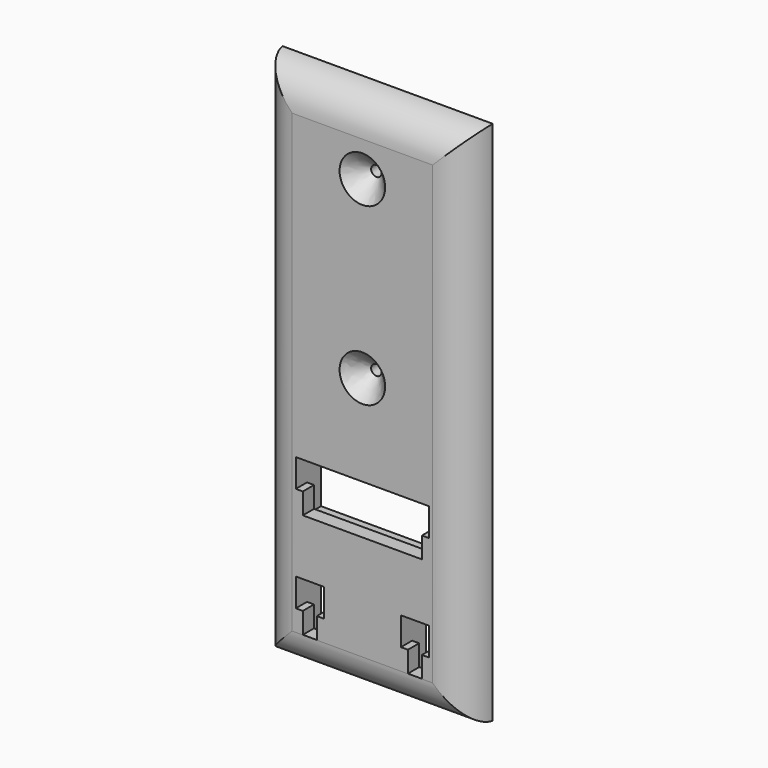
from build123d import *
from build123d import SkipClean  # not in build123d's __all__

# Parameters (mm, degrees)
F0_R        = 1.5
F1_DEPTH    = 5
F0_W        = 22
F0_H        = 2
F0_W_2      = 2
F0_H_2      = 6
F0_W_3      = 4
F2_DEPTH    = 4
F3_SIZE     = 5
F4_T1_DEPTH = 109.7493718553
F4_T3_DEPTH = 199.7493718553


# Not quite as in the source:
# - a fillet or chamfer that OpenCascade refuses, or shapes differently, is made with other operations: its cross-section is extruded or revolved along the edge and cut away or added
# - a feature names something its author has since deleted; it is built from what else it names


with BuildPart() as f1:
    # F0 (on Front) → F1 (new body)
    with BuildSketch(Plane.XZ):
        with BuildLine():
            Line((-30, 150), (-30, 80))
            Line((-30, 80), (-1.5, 80))
            ThreePointArc((-1.5, 80), (0, 81.5), (1.5, 80))
            Line((1.5, 80), (30, 80))
            Line((30, 80), (30, 150))
            Line((30, 150), (-30, 150))
        make_face()
        with Locations((0, 130)):
            Circle(F0_R, mode=Mode.SUBTRACT)
        with BuildLine():
            Line((-30, 0), (0, 0))
            Line((0, 0), (30, 0))
            Line((30, 0), (30, 80))
            Line((30, 80), (1.5, 80))
            ThreePointArc((1.5, 80), (0, 78.5), (-1.5, 80))
            Line((-1.5, 80), (-30, 80))
            Line((-30, 80), (-30, 0))
        make_face()
        Polygon((-11, 24), (-11, 16), (-11, 10), (-11, 8), (-13, 8), (-17, 8), (-19, 8), (-19, 10), (-19, 16), (-19, 24), align=None, mode=Mode.SUBTRACT)
        Polygon((19, 24), (19, 16), (19, 10), (19, 8), (17, 8), (13, 8), (11, 8), (11, 10), (11, 16), (11, 24), align=None, mode=Mode.SUBTRACT)
        Polygon((-19, 54), (-11, 54), (11, 54), (19, 54), (19, 46), (19, 40), (19, 38), (17, 38), (13, 38), (11, 38), (-11, 38), (-13, 38), (-17, 38), (-19, 38), (-19, 40), (-19, 46), (-19, 48), align=None, mode=Mode.SUBTRACT)
    extrude(amount=-F1_DEPTH)

    # F0 (on Front) → F2 (join)
    with BuildSketch(Plane.XZ):
        with BuildLine():
            Line((-30, 0), (0, 0))
            Line((0, 0), (30, 0))
            Line((30, 0), (30, 80))
            Line((30, 80), (1.5, 80))
            ThreePointArc((1.5, 80), (0, 78.5), (-1.5, 80))
            Line((-1.5, 80), (-30, 80))
            Line((-30, 80), (-30, 0))
        make_face()
        Polygon((-11, 24), (-11, 16), (-11, 10), (-11, 8), (-13, 8), (-17, 8), (-19, 8), (-19, 10), (-19, 16), (-19, 24), align=None, mode=Mode.SUBTRACT)
        Polygon((19, 24), (19, 16), (19, 10), (19, 8), (17, 8), (13, 8), (11, 8), (11, 10), (11, 16), (11, 24), align=None, mode=Mode.SUBTRACT)
        Polygon((-19, 54), (-11, 54), (11, 54), (19, 54), (19, 46), (19, 40), (19, 38), (17, 38), (13, 38), (11, 38), (-11, 38), (-13, 38), (-17, 38), (-19, 38), (-19, 40), (-19, 46), (-19, 48), align=None, mode=Mode.SUBTRACT)
        with BuildLine():
            Line((-30, 150), (-30, 80))
            Line((-30, 80), (-1.5, 80))
            ThreePointArc((-1.5, 80), (0, 81.5), (1.5, 80))
            Line((1.5, 80), (30, 80))
            Line((30, 80), (30, 150))
            Line((30, 150), (-30, 150))
        make_face()
        with Locations((0, 130)):
            Circle(F0_R, mode=Mode.SUBTRACT)
        with Locations((0, 39)):
            Rectangle(F0_W, F0_H)
        with Locations((-18, 43)):
            Rectangle(F0_W_2, F0_H_2)
        with Locations((18, 43)):
            Rectangle(F0_W_2, F0_H_2)
        with Locations((-18, 13)):
            Rectangle(F0_W_2, F0_H_2)
        with Locations((-12, 13)):
            Rectangle(F0_W_2, F0_H_2)
        with Locations((12, 13)):
            Rectangle(F0_W_2, F0_H_2)
        with Locations((18, 13)):
            Rectangle(F0_W_2, F0_H_2)
        with Locations((-15, 39)):
            Rectangle(F0_W_3, F0_H)
        with Locations((15, 39)):
            Rectangle(F0_W_3, F0_H)
        with Locations((-15, 9)):
            Rectangle(F0_W_3, F0_H)
        with Locations((15, 9)):
            Rectangle(F0_W_3, F0_H)
        with Locations((-18, 39)):
            Rectangle(F0_W_2, F0_H)
        with Locations((-12, 39)):
            Rectangle(F0_W_2, F0_H)
        with Locations((12, 39)):
            Rectangle(F0_W_2, F0_H)
        with Locations((18, 39)):
            Rectangle(F0_W_2, F0_H)
        with Locations((-18, 9)):
            Rectangle(F0_W_2, F0_H)
        with Locations((-12, 9)):
            Rectangle(F0_W_2, F0_H)
        with Locations((12, 9)):
            Rectangle(F0_W_2, F0_H)
        with Locations((18, 9)):
            Rectangle(F0_W_2, F0_H)
    with SkipClean():  # cleaning this boolean's faces spoils the solid; the shape is the same uncleaned
        extrude(amount=F2_DEPTH)

    # F3
    f3_edges = [f1.edges().sort_by_distance(p)[0] for p in [
        (-1.5, -4, 130),
        (1.5, -4, 80),
    ]]
    chamfer(f3_edges, length=F3_SIZE)

    # F4: fillet of radius 10 on 4 edges, made by hand

    # F4_s2 → F4_t1 (cut)
    with BuildSketch(Plane.YZ.offset(-54.8746859277)):
        with BuildLine():
            ThreePointArc((-4, 9.9498743711), (-1.4161984871, 3.2416704386), (5, 0))
            Line((5, 0), (-4, 0))
            Line((-4, 0), (-4, 9.9498743711))
        make_face()
        with BuildLine():
            ThreePointArc((-4, 140.0501256289), (-1.4161984871, 146.7583295614), (5, 150))
            Line((5, 150), (-4, 150))
            Line((-4, 150), (-4, 140.0501256289))
        make_face()
    extrude(amount=F4_T1_DEPTH, mode=Mode.SUBTRACT)

    # F4_s4 → F4_t3 (cut)
    with BuildSketch(Plane.XY.offset(-24.8746859277)):
        with BuildLine():
            ThreePointArc((-20.0501256289, -4), (-26.7583295614, -1.4161984871), (-30, 5))
            Line((-30, 5), (-30, -4))
            Line((-30, -4), (-20.0501256289, -4))
        make_face()
        with BuildLine():
            ThreePointArc((20.0501256289, -4), (26.7583295614, -1.4161984871), (30, 5))
            Line((30, 5), (30, -4))
            Line((30, -4), (20.0501256289, -4))
        make_face()
    extrude(amount=F4_T3_DEPTH, mode=Mode.SUBTRACT)


solid = f1.part
